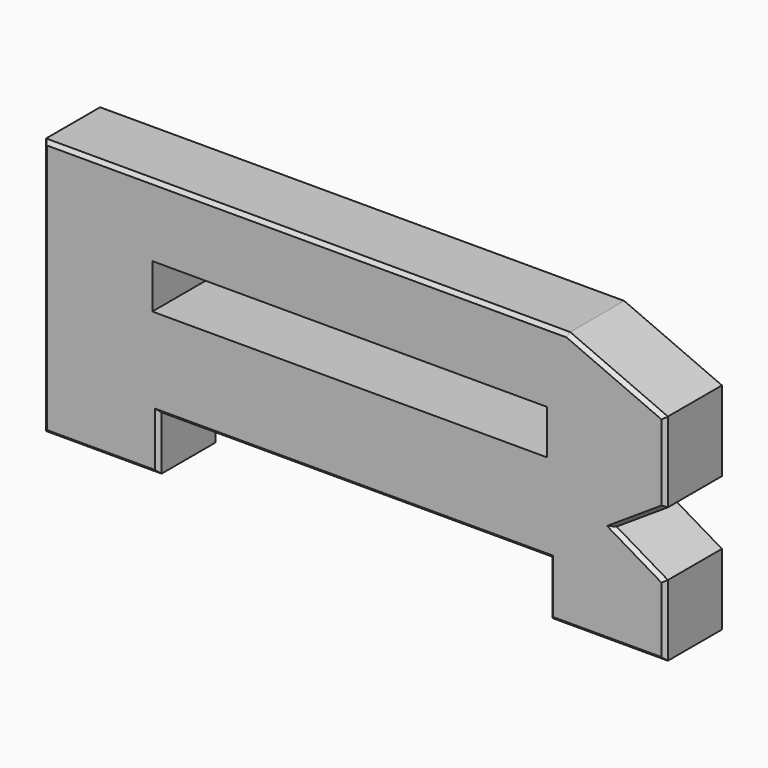
from build123d import *

# Parameters (mm, degrees)
F0_W         = 141.1362439394
F0_H         = 15.875
F1_DEPTH     = 25.4
F2_SIZE      = 1.27
F3_T         = 3.81
F3_T3_DEPTH  = 31.75
F3_T5_DEPTH  = 10.3365589148
F3_T7_DEPTH  = 33.02
F3_T9_DEPTH  = 9.8197045256
F3_T11_DEPTH = 9.8197045256
F4_R         = 4.1275
F4_R_2       = 1.8415
F5_DEPTH     = 21.59


# Not quite as in the source:
# - a shell that OpenCascade refuses in one call is made with other operations: the cavity is built on its own and cut out
# - a feature names something its author has since deleted; it is built from what else it names


with BuildPart() as f1:
    # F0 (on Front) → F1 (new body)
    with BuildSketch(Plane.XZ):
        Polygon((115.6852519128, 43.8017650865), (-71.6397480872, 43.8017650865), (-71.6397480872, -48.2732349135), (-30.3647480872, -48.2732349135), (-30.3647480872, -28.973974956), (109.3352519128, -28.973974956), (109.3352519128, -48.2732349135), (150.6102519128, -48.2732349135), (150.6102519128, -22.8732349135), (132.2698407767, -12.0163811026), (150.6102519128, 0), (150.6102519128, 28.575), align=None)
        with Locations((37.9095822573, 10.4642650865)):
            Rectangle(F0_W, F0_H, mode=Mode.SUBTRACT)
    extrude(amount=F1_DEPTH)

    # F2
    f2_edges = [f1.edges().sort_by_distance(p)[0] for p in [
        (-71.639748, -25.4, -2.235735),
        (22.022752, -25.4, 43.801765),
        (133.147752, -25.4, 36.188383),
        (150.610252, -25.4, 14.2875),
        (141.440046, -25.4, -6.008191),
        (141.440046, -25.4, -17.444808),
        (150.610252, -25.4, -35.573235),
        (129.972752, -25.4, -48.273235),
        (109.335252, -25.4, -38.623605),
        (39.485252, -25.4, -28.973975),
        (-30.364748, -25.4, -38.623605),
        (-51.002248, -25.4, -48.273235),
    ]]
    chamfer(f2_edges, length=F2_SIZE)

    # F3: shell of thickness 3.81, made by hand


with BuildPart() as f3_core1:
    # F3_t2: copy of F1
    add(f1.part)

    # the walls: a layer under each face that stays
    f3_faces = [f3_core1.faces().sort_by_distance(p)[0] for p in [
        (141.4400463447, -12.065, -17.4448080081),
        (150.6102519128, -12.065, -35.5732349135),
        (140.2396500387, -24.765, -17.4721355193),
        (141.4400463447, -12.065, -6.0081905513),
        (129.9727519128, -12.065, -48.2732349135),
        (149.9752519128, -24.765, -35.5732349135),
        (39.4852519128, -25.4, -2.2357349135),
        (140.2396500387, -24.765, -6.0355180626),
        (150.6102519128, -12.065, 14.2875),
        (133.1477519128, -12.065, 36.1883825433),
        (22.0227519128, -12.065, 43.8017650865),
        (-71.6397480872, -12.065, -2.2357349135),
        (-51.0022480872, -12.065, -48.2732349135),
        (-30.3647480872, -12.065, -38.6236049347),
        (39.4852519128, -12.065, -28.973974956),
        (109.3352519128, -12.065, -38.6236049347),
        (-32.6585397124, -12.7, 10.4642650865),
        (37.9095822573, -12.7, 18.4017650865),
        (108.477704227, -12.7, 10.4642650865),
        (37.9095822573, -12.7, 2.5267650865),
        (129.9727519128, -24.765, -47.6382349135),
        (-71.0047480872, -24.765, -2.2357349135),
        (22.0227519128, -24.765, 43.1667650865),
        (-51.0022480872, -24.765, -47.6382349135),
        (132.8939724947, -24.765, 35.6062992099),
        (-30.9997480872, -24.765, -37.9886049347),
        (149.9752519128, -24.765, 14.2875),
        (39.4852519128, -24.765, -28.338974956),
        (109.9702519128, -24.765, -37.9886049347),
    ]]
    thicken(f3_faces, amount=-F3_T, mode=Mode.SUBTRACT)

    # F3_s4 → F3_t3 (cut)
    with BuildSketch(Plane.XZ.offset(-3.81)):
        Polygon((132.3101290844, -12.0154639229), (130.3290203992, -15.2949960941), (125.0674629404, -12.1803461703), (130.1818303825, -8.8294840861), align=None)
        Polygon((-30.3266480872, -29.012074956), (-34.1747480872, -28.973974956), (-34.1747480872, -25.163974956), (-30.3647480872, -25.163974956), align=None)
        Polygon((109.2971519128, -29.012074956), (109.3352519128, -25.163974956), (113.1452519128, -25.163974956), (113.1452519128, -28.973974956), align=None)
    extrude(amount=F3_T3_DEPTH, mode=Mode.SUBTRACT)

    # F3_s6 → F3_t5 (cut)
    with BuildSketch(Plane(origin=(96.491386595, 51.0431681427, 2.1966657526), x_dir=(0.4675978526, -0.8839413149, 0), z_dir=(-0.8837623948, -0.4675032053, -0.0201192112))):
        Polygon((83.2395465479, -14.1386059374), (80.1554756401, -16.4580548587), (78.415785798, -14.1899447458), (80.1068084957, -11.8853218988), align=None)
    extrude(amount=F3_T5_DEPTH, mode=Mode.SUBTRACT)

    # F3_s8 → F3_t7 (cut)
    with BuildSketch(Plane.XZ.offset(-3.81)):
        Polygon((-32.6204397124, 2.5648650865), (-36.4685397124, 2.5267650865), (-36.4685397124, -1.2832349135), (-32.6585397124, -1.2832349135), align=None)
        Polygon((-32.6204397124, 18.3636650865), (-36.4685397124, 18.4017650865), (-36.4685397124, 22.2117650865), (-32.6585397124, 22.2117650865), align=None)
        Polygon((108.439604227, 18.3636650865), (108.477704227, 22.2117650865), (112.287704227, 22.2117650865), (112.287704227, 18.4017650865), align=None)
        Polygon((108.439604227, 2.5648650865), (112.287704227, 2.5267650865), (112.287704227, -1.2832349135), (108.477704227, -1.2832349135), align=None)
    extrude(amount=F3_T7_DEPTH, mode=Mode.SUBTRACT)

    # F3_s10 → F3_t9 (cut)
    with BuildSketch(Plane(origin=(-6.3072198515, -6.3072198515, 6.3072198515), x_dir=(0.7071067812, -0.7071067812, 0), z_dir=(-0.5773502692, -0.5773502692, 0.5773502692))):
        Polygon((-4.3514826515, -45.9375348012), (-8.2186326515, -45.9045392333), (-8.2186326515, -43.7048347077), (-6.3136326515, -42.6049824449), align=None)
    extrude(amount=F3_T9_DEPTH, mode=Mode.SUBTRACT)

    # F3_s12 → F3_t11 (cut)
    with BuildSketch(Plane(origin=(32.6307211267, -32.6307211267, 32.6307211267), x_dir=(0.7071067812, 0.7071067812, 0), z_dir=(0.5773502692, -0.5773502692, 0.5773502692))):
        Polygon((60.1920614202, -78.177107985), (62.1542114202, -74.8445556287), (64.0592114202, -75.9444078915), (64.0592114202, -78.1441124172), align=None)
    extrude(amount=F3_T11_DEPTH, mode=Mode.SUBTRACT)


with BuildPart() as f1_1:
    add(f1.part)

    # what is left inside the walls is the cavity
    f3_cavity = [f3_core1.part.solids().sort_by_distance(p)[0] for p in [
        (39.485252, -21.5519, -16.311568),
    ]]
    add(f3_cavity, mode=Mode.SUBTRACT)

    # F4 (on face) → F5 (join, through all)
    with BuildSketch(Plane(origin=(0, -21.59, 0), x_dir=(-1, 0, 0), z_dir=(0, 1, 0))):
        with Locations((48.7797480872, 21.8307650865)):
            Circle(F4_R)
        with Locations((48.7797480872, 21.8307650865)):
            Circle(F4_R_2, mode=Mode.SUBTRACT)
        with Locations((48.7797480872, -28.8422349135)):
            Circle(F4_R)
        with Locations((48.7797480872, -28.8422349135)):
            Circle(F4_R_2, mode=Mode.SUBTRACT)
        with Locations((-125.7182519128, 19.8926216617)):
            Circle(F4_R)
        with Locations((-125.7182519128, 19.8926216617)):
            Circle(F4_R_2, mode=Mode.SUBTRACT)
        with Locations((-125.7182519128, -31.1790349135)):
            Circle(F4_R)
        with Locations((-125.7182519128, -31.1790349135)):
            Circle(F4_R_2, mode=Mode.SUBTRACT)
    extrude(amount=F5_DEPTH)


solid = f1_1.part
